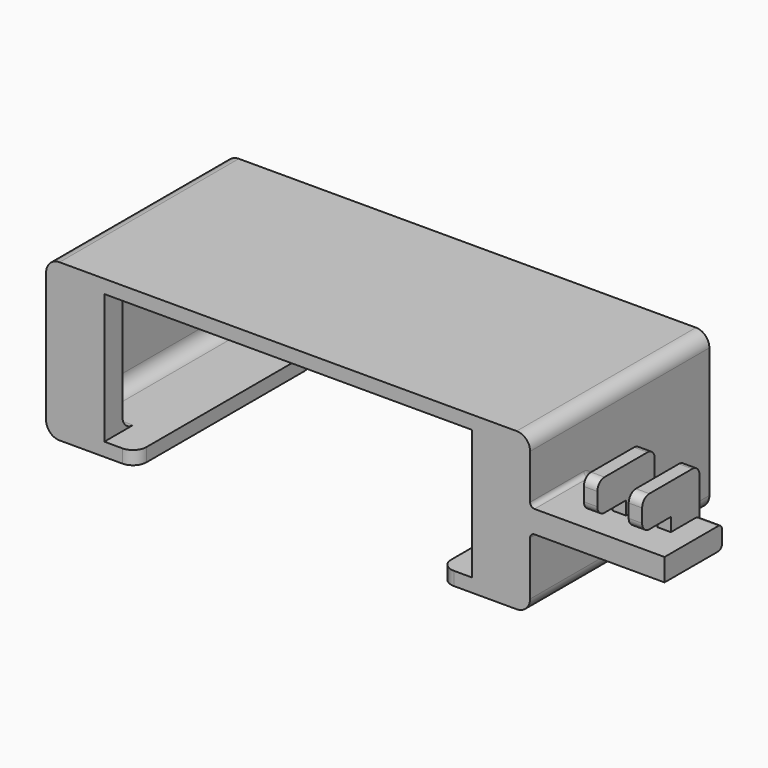
from build123d import *

# Parameters (mm, degrees)
F0_W     = 3
F0_H     = 16
F1_DEPTH = 10
F2_W     = 8
F2_H     = 3
F3_DEPTH = 25
F4_W     = 30
F4_H     = 16
F5_DEPTH = 5
F7_DEPTH = 50
F6_W     = 10
F6_H     = 29
F8_DEPTH = 5
F9_R     = 2
F10_R    = 3
F11_R    = 1


with BuildPart() as f1:
    # F0 (on Top) → F1 (new body)
    with BuildSketch(Plane.XY):
        with Locations((-5, 8)):
            Rectangle(F0_W, F0_H)
    extrude(amount=F1_DEPTH)


with BuildPart() as f1b:
    # F0 (on Top) → F1, piece 2 (new body)
    with BuildSketch(Plane.XY):
        with Locations((5, 8)):
            Rectangle(F0_W, F0_H)
    extrude(amount=F1_DEPTH)


with BuildPart() as f3_tool:
    # F2 (on face) → F3 (new body)
    with BuildSketch(Plane(origin=(-6.5, 0, 0), x_dir=(0, -1, 0), z_dir=(-1, 0, 0))):
        with Locations((-4, 1.5)):
            Rectangle(F2_W, F2_H)
    extrude(amount=-F3_DEPTH)


with BuildPart() as f1_1:
    add(f1.part)

    # F3: cut by f3_tool
    add(f3_tool.part, mode=Mode.SUBTRACT)



with BuildPart() as f1b_1:
    add(f1b.part)

    # F3: cut by f3_tool
    add(f3_tool.part, mode=Mode.SUBTRACT)


with BuildPart() as f1_2:
    add(f1_1.part)

    add(f1b_1.part)  # F5 merges F1b
    # F4 (on Top) → F5 (join)
    with BuildSketch(Plane.XY):
        with Locations((-3.5, 8)):
            Rectangle(F4_W, F4_H)
    extrude(amount=-F5_DEPTH)

    # F6 (on Front) → F7 (join)
    with BuildSketch(Plane.XZ):
        Polygon((-113.5, -18), (-123.5, -18), (-123.5, 11), (-113.5, 11), (-31.5, 11), (-21.5, 11), (-21.5, -18), (-31.5, -18), (-38.5, -18), (-38.5, -21), (-18.5, -21), (-18.5, 14), (-126.5, 14), (-126.5, -21), (-106.5, -21), (-106.5, -18), align=None)
    extrude(amount=-F7_DEPTH)

    # F6 (on Front) → F8 (join)
    with BuildSketch(Plane.XZ):
        with Locations((-26.5, -3.5)):
            Rectangle(F6_W, F6_H)
        with Locations((-118.5, -3.5)):
            Rectangle(F6_W, F6_H)
    extrude(amount=-F8_DEPTH)

    # F9
    f9_edges = [f1_2.edges().sort_by_distance(p)[0] for p in [
        (-5, 16, 10),
        (5, 16, 10),
        (-5, 0, 10),
        (5, 0, 10),
        (-5, 0, 3),
        (5, 0, 3),
    ]]
    fillet(f9_edges, radius=F9_R)

    # F10
    f10_edges = [f1_2.edges().sort_by_distance(p)[0] for p in [
        (-21.5, 27.5, 11),
        (-123.5, 27.5, 11),
        (-126.5, 25, 14),
        (-18.5, 25, 14),
        (-18.5, 25, -21),
        (-21.5, 27.5, -18),
        (-123.5, 27.5, -18),
        (-126.5, 25, -21),
        (-123.5, 5, -3.5),
        (-118.5, 5, -18),
        (-26.5, 5, -18),
        (-21.5, 5, -3.5),
        (-26.5, 5, 11),
        (-118.5, 5, 11),
        (-38.5, 0, -19.5),
        (-106.5, 0, -19.5),
        (-38.5, 50, -19.5),
        (-106.5, 50, -19.5),
    ]]
    fillet(f10_edges, radius=F10_R)

    # F11
    f11_edges = [f1_2.edges().sort_by_distance(p)[0] for p in [
        (-18.5, 16, -2.5),
        (-3.5, 16, -5),
        (-12.5, 16, 0),
        (0, 16, 0),
        (9, 16, 0),
        (-18.5, 8, -5),
        (-18.5, 8, 0),
    ]]
    fillet(f11_edges, radius=F11_R)


solid = f1_2.part
